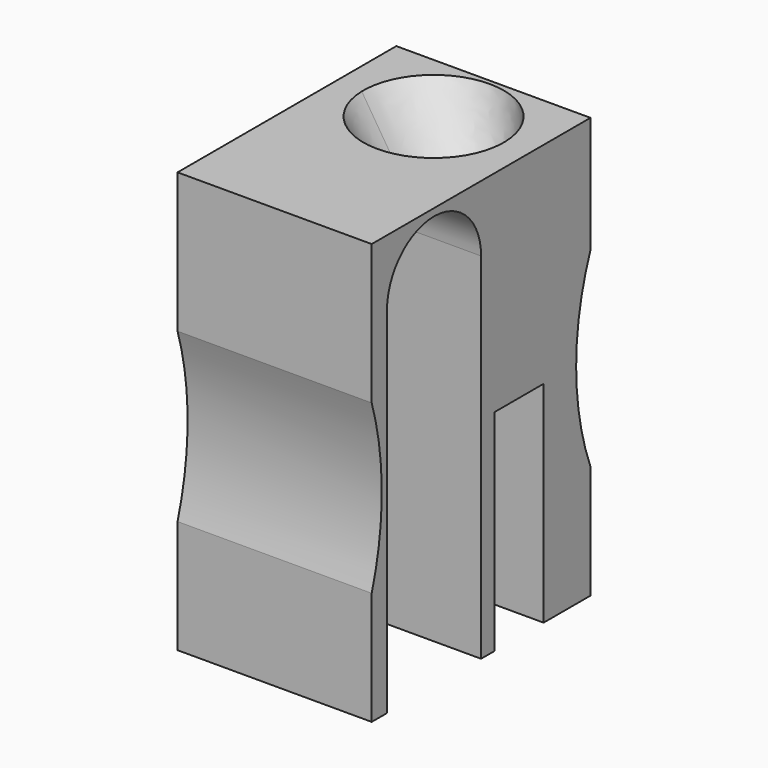
from build123d import *

# Parameters (mm, degrees)
F0_W      = 16.9
F0_H      = 26
F1_DEPTH  = 6
F4_DEPTH  = 8
F7_DEPTH  = 13
F13_R     = 1.0372867361
F14_DEPTH = 3
F16_DEPTH = 12


# Not quite as in the source:
# - the arcs of a loft's sections are written as splines that run evenly, so that the points pair up as in the source's solid


with BuildPart() as f1:
    # F0 (on Right) → F1 (new body, symmetric)
    with BuildSketch(Plane.YZ):
        Rectangle(F0_W, F0_H)
    extrude(amount=F1_DEPTH, both=True)

    # F3 (on offset) → F4 (cut)
    with BuildSketch(Plane.YZ.offset(6)):
        with BuildLine():
            Line((0, -13.1401689723), (0, 0))
            Line((0, 0), (0, 8.9160166681))
            ThreePointArc((0, 8.9160166681), (-3.6351196468, 12.5511363149), (-7.2702392936, 8.9160166681))
            Line((-7.2702392936, 8.9160166681), (-7.2702392936, 0))
            Line((-7.2702392936, 0), (-7.2702392936, -13.1401689723))
            Line((-7.2702392936, -13.1401689723), (0, -13.1401689723))
        make_face()
    extrude(amount=-F4_DEPTH, mode=Mode.SUBTRACT)

    # F6 (on offset) → F7 (cut)
    with BuildSketch(Plane.XY.offset(-13)):
        with BuildLine():
            Line((0, 1.0551682208), (6, 1.0551682208))
            Line((6, 1.0551682208), (6, 4.8324568197))
            Line((6, 4.8324568197), (0, 4.8324568197))
            ThreePointArc((0, 4.8324568197), (-1.8886442995, 2.9438125202), (0, 1.0551682208))
        make_face()
    extrude(amount=F7_DEPTH, mode=Mode.SUBTRACT)

    # F10 (on offset) → F11 section 0
    with BuildSketch(Plane.XY.offset(13)):
        with BuildLine():
            add(Edge.make_bspline(
                [(4.3429478235, 3.9498277403), (4.3273258404, 4.518318281), (4.1986746967, 5.0834789619), (3.734705213, 6.1219559637), (3.3995694252, 6.5948636881), (2.5735095721, 7.3767379005), (2.0829105259, 7.6853967543), (1.0205204277, 8.0916349162), (0.4491473807, 8.1890543869), (-0.6878337007, 8.1578104207), (-1.2529943817, 8.0291592769), (-2.2914713834, 7.5651897932), (-2.7643791079, 7.2300540055), (-3.5462533203, 6.4039941523), (-3.8549121741, 5.9133951062), (-4.261150336, 4.8510050079), (-4.3585698066, 4.279631961), (-4.3429478235, 3.7111414202)],
                knots=[0, 0, 0, 0, 0.125, 0.125, 0.25, 0.25, 0.375, 0.375, 0.5, 0.5, 0.625, 0.625, 0.75, 0.75, 0.875, 0.875, 1, 1, 1, 1], degree=3))
            add(Edge.make_bspline(
                [(-4.3429478235, 3.7111414202), (-4.3273258404, 3.1426508795), (-4.1986746967, 2.5774901986), (-3.734705213, 1.5390131968), (-3.3995694252, 1.0661054724), (-2.5735095721, 0.28423126), (-2.0829105259, -0.0244275938), (-1.0205204277, -0.4306657557), (-0.4491473807, -0.5280852264), (0.6878337007, -0.4968412602), (1.2529943817, -0.3681901164), (2.2914713834, 0.0957793673), (2.7643791079, 0.430915155), (3.5462533203, 1.2569750082), (3.8549121741, 1.7475740543), (4.261150336, 2.8099641525), (4.3585698066, 3.3813371995), (4.3429478235, 3.9498277403)],
                knots=[0, 0, 0, 0, 0.125, 0.125, 0.25, 0.25, 0.375, 0.375, 0.5, 0.5, 0.625, 0.625, 0.75, 0.75, 0.875, 0.875, 1, 1, 1, 1], degree=3))
        make_face()
    # F8 (on Top) → F11 section 1
    with BuildSketch(Plane.XY):
        with BuildLine():
            Line((6, 1.9599355292), (6, 3.9953631349))
            add(Edge.make_bspline(
                [(6, 3.9953631349), (5.8728482854, 4.0351535262), (5.7381950052, 4.0508266131), (5.4724119576, 4.0317817528), (5.3413690344, 3.9970700285), (5.1010102922, 3.8820439003), (4.9917730101, 3.8017670809), (4.8102123375, 3.6067310401), (4.7379482715, 3.4920355462), (4.640395332, 3.2440703086), (4.6151383336, 3.110881587), (4.6151383336, 2.844417077), (4.640395332, 2.7112283554), (4.7379482715, 2.4632631178), (4.8102123375, 2.348567624), (4.9917730101, 2.1535315831), (5.1010102922, 2.0732547638), (5.3413690344, 1.9582286356), (5.4724119576, 1.9235169113), (5.7381950052, 1.904472051), (5.8728482854, 1.9201451378), (6, 1.9599355292)],
                knots=[0, 0, 0, 0, 0.1, 0.1, 0.2, 0.2, 0.3, 0.3, 0.4, 0.4, 0.5, 0.5, 0.6, 0.6, 0.7, 0.7, 0.8, 0.8, 0.9, 0.9, 1, 1, 1, 1], degree=3))
        make_face()
    loft(ruled=True, mode=Mode.SUBTRACT)

    # F13 (on offset) → F14 (cut)
    with BuildSketch(Plane.YZ.offset(-2)):
        with Locations((-4.3216282502, 0)):
            Circle(F13_R)
    extrude(amount=-F14_DEPTH, mode=Mode.SUBTRACT)

    # F15 (on offset) → F16 (cut)
    with BuildSketch(Plane.YZ.offset(6)):
        with BuildLine():
            Line((8.45, -5.9837657027), (8.45, 5.8088130318))
            ThreePointArc((8.45, 5.8088130318), (7.3449803731, -0.0874763355), (8.45, -5.9837657027))
        make_face()
        with BuildLine():
            Line((-8.45, 4.3591358699), (-8.45, -5.9991455637))
            ThreePointArc((-8.45, -5.9991455637), (-7.6726197795, -0.8200048469), (-8.45, 4.3591358699))
        make_face()
    extrude(amount=-F16_DEPTH, mode=Mode.SUBTRACT)


solid = f1.part
